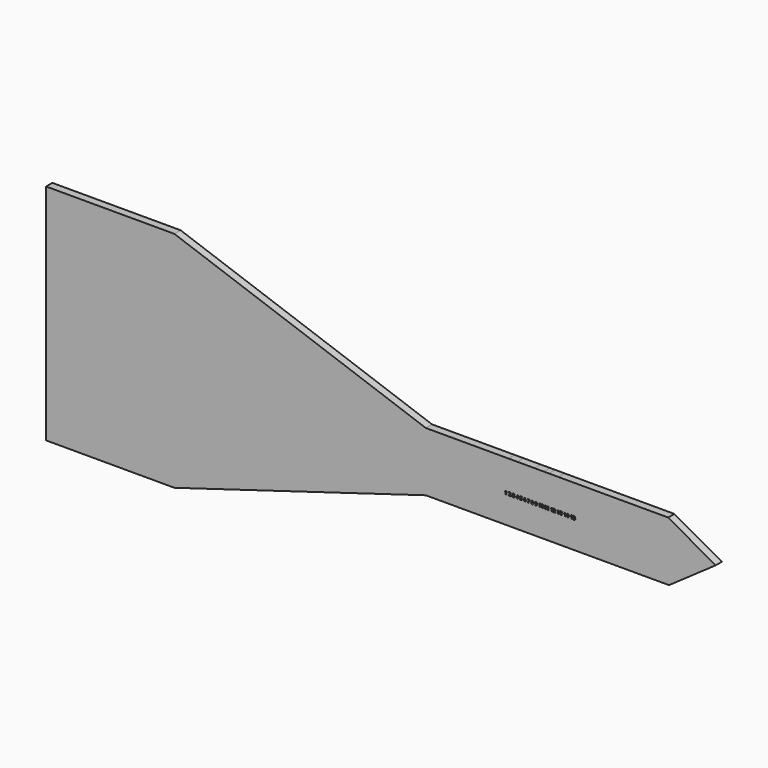
from build123d import *

# Parameters (mm, degrees)
F1_DEPTH = 1.42748
F7_DEPTH = 1.42748
F0_W     = 0.7037650794
F0_H     = 10.8203962445
F0_W_2   = 0.7917359471
F0_W_3   = 0.9236931801
F8_DEPTH = 1.42748


# Not quite as in the source:
# - the program builds the solid bodies; features that only make, move or delete a surface that nothing else refers to are left out


with BuildPart() as f1:
    # F0 (on Front) → F1 (new body)
    with BuildSketch(Plane.XZ):
        Polygon((0, 29.5358654112), (-45.9049940109, 45.8104424179), (-69.3307071924, 45.8104424179), (-69.3307071924, 4.9920389429), (-45.9049940109, 4.9920389429), (0, 18.7154691666), (14.3839064986, 18.7154691666), (14.3839064986, 29.5358654112), align=None)
    extrude(amount=F1_DEPTH)


with BuildPart() as f7:
    # F0 (on Front) → F7 (new body)
    with BuildSketch(Plane.XZ):
        Polygon((44.2517474294, 29.5358654112), (27.3507699184, 29.5358654112), (27.3507699184, 18.7154691666), (44.4178134203, 18.7154691666), (52.930470556, 24.6695391834), align=None)
    extrude(amount=F7_DEPTH)


with BuildPart() as f8:
    # F0 (on Front) → F8 (new body)
    with BuildSketch(Plane.XZ):
        Polygon((0, 29.5358654112), (-45.9049940109, 45.8104424179), (-69.3307071924, 45.8104424179), (-69.3307071924, 4.9920389429), (-45.9049940109, 4.9920389429), (0, 18.7154691666), (14.3839064986, 18.7154691666), (14.3839064986, 29.5358654112), align=None)
        with Locations((14.7357890382, 24.1256672889)):
            Rectangle(F0_W, F0_H)
        with BuildLine():
            Line((14.7264703071, 24.1856664079), (14.7264703071, 23.5936943802))
            Line((14.7264703071, 23.5936943802), (14.601312728, 23.5936943802))
            Line((14.601312728, 23.5936943802), (14.601312728, 23.9362581887))
            Line((14.601312728, 23.9362581887), (14.6026083551, 23.9924884054))
            Line((14.6026083551, 23.9924884054), (14.6045517958, 24.0540306932))
            add(Edge.make_bspline(
                [(14.6045517958, 24.0540306932), (14.5734567451, 24.0229356425), (14.5612778502, 24.0132184392)],
                knots=[0, 0, 0, 1, 1, 1], degree=2))
            Line((14.5612778502, 24.0132184392), (14.4932574268, 23.9585429751))
            Line((14.4932574268, 23.9585429751), (14.4328812034, 24.0338189103))
            Line((14.4328812034, 24.0338189103), (14.6235975144, 24.1856664079))
            Line((14.6235975144, 24.1856664079), (14.7264703071, 24.1856664079))
        make_face(mode=Mode.SUBTRACT)
        with BuildLine():
            Line((15.8354230225, 29.5358654112), (15.0876715779, 29.5358654112))
            Line((15.0876715779, 29.5358654112), (15.0876715779, 18.7154691666))
            Line((15.0876715779, 18.7154691666), (15.8354230225, 18.7154691666))
            Line((15.8354230225, 18.7154691666), (15.8354230225, 23.6024215287))
            add(Edge.make_bspline(
                [(15.8354230225, 23.6024215287), (15.8134077009, 23.6087806021), (15.793030546, 23.6175339191)],
                knots=[0.7264758514, 0.7264758514, 0.7264758514, 1, 1, 1], degree=2))
            Line((15.793030546, 23.6175339191), (15.793030546, 23.7240344677))
            add(Edge.make_bspline(
                [(15.793030546, 23.7240344677), (15.8130388008, 23.7139170861), (15.8354230225, 23.7059776741)],
                knots=[0, 0, 0, 0.5827513749, 0.5827513749, 0.5827513749], degree=2))
            Line((15.8354230225, 23.7059776741), (15.8354230225, 24.0738741563))
            Line((15.8354230225, 24.0738741563), (15.7938079223, 24.135784764))
            add(Edge.make_bspline(
                [(15.7938079223, 24.135784764), (15.8136756548, 24.1500895314), (15.8354230225, 24.1608846064)],
                knots=[0, 0, 0, 0.2453512407, 0.2453512407, 0.2453512407], degree=2))
            Line((15.8354230225, 24.1608846064), (15.8354230225, 29.5358654112))
        make_face()
        with BuildLine():
            Line((15.5196532253, 23.6990288644), (15.5196532253, 23.5936943802))
            Line((15.5196532253, 23.5936943802), (15.1058299256, 23.5936943802))
            Line((15.1058299256, 23.5936943802), (15.1058299256, 23.6807605222))
            Line((15.1058299256, 23.6807605222), (15.2544383554, 23.8309237045))
            add(Edge.make_bspline(
                [(15.2544383554, 23.8309237045), (15.3205153381, 23.8985554398), (15.3407271211, 23.9246623261)],
                knots=[0, 0, 0, 1, 1, 1], degree=2))
            add(Edge.make_bspline(
                [(15.3407271211, 23.9246623261), (15.360938904, 23.9507692124), (15.3698787311, 23.9730539987)],
                knots=[0, 0, 0, 1, 1, 1], degree=2))
            add(Edge.make_bspline(
                [(15.3698787311, 23.9730539987), (15.3788185582, 23.9953387851), (15.3788185582, 24.0191783239)],
                knots=[0, 0, 0, 1, 1, 1], degree=2))
            add(Edge.make_bspline(
                [(15.3788185582, 24.0191783239), (15.3788185582, 24.0548080695), (15.3591250261, 24.0722342542)],
                knots=[0, 0, 0, 1, 1, 1], degree=2))
            add(Edge.make_bspline(
                [(15.3591250261, 24.0722342542), (15.339431494, 24.0896604388), (15.306652128, 24.0896604388)],
                knots=[0, 0, 0, 1, 1, 1], degree=2))
            add(Edge.make_bspline(
                [(15.306652128, 24.0896604388), (15.2723180095, 24.0896604388), (15.2399273317, 24.0738537881)],
                knots=[0, 0, 0, 1, 1, 1], degree=2))
            add(Edge.make_bspline(
                [(15.2399273317, 24.0738537881), (15.2075366539, 24.0580471373), (15.1722955965, 24.0288955273)],
                knots=[0, 0, 0, 1, 1, 1], degree=2))
            Line((15.1722955965, 24.0288955273), (15.1042751731, 24.1094835337))
            add(Edge.make_bspline(
                [(15.1042751731, 24.1094835337), (15.1479378067, 24.1467975945), (15.1767007286, 24.1621507758)],
                knots=[0, 0, 0, 1, 1, 1], degree=2))
            add(Edge.make_bspline(
                [(15.1767007286, 24.1621507758), (15.2054636505, 24.1775039571), (15.2394738622, 24.1857959706)],
                knots=[0, 0, 0, 1, 1, 1], degree=2))
            add(Edge.make_bspline(
                [(15.2394738622, 24.1857959706), (15.2734840739, 24.1940879841), (15.3155919551, 24.1940879841)],
                knots=[0, 0, 0, 1, 1, 1], degree=2))
            add(Edge.make_bspline(
                [(15.3155919551, 24.1940879841), (15.3710447955, 24.1940879841), (15.4135413648, 24.1738762011)],
                knots=[0, 0, 0, 1, 1, 1], degree=2))
            add(Edge.make_bspline(
                [(15.4135413648, 24.1738762011), (15.4560379341, 24.1536644182), (15.4795535662, 24.117192515)],
                knots=[0, 0, 0, 1, 1, 1], degree=2))
            add(Edge.make_bspline(
                [(15.4795535662, 24.117192515), (15.5030691983, 24.0807206118), (15.5030691983, 24.0338189103)],
                knots=[0, 0, 0, 1, 1, 1], degree=2))
            add(Edge.make_bspline(
                [(15.5030691983, 24.0338189103), (15.5030691983, 23.9928770935), (15.4886877373, 23.9570530039)],
                knots=[0, 0, 0, 1, 1, 1], degree=2))
            add(Edge.make_bspline(
                [(15.4886877373, 23.9570530039), (15.4743062764, 23.9212289142), (15.4441181646, 23.8835909466)],
                knots=[0, 0, 0, 1, 1, 1], degree=2))
            add(Edge.make_bspline(
                [(15.4441181646, 23.8835909466), (15.4139300529, 23.845952979), (15.3378767414, 23.7762482403)],
                knots=[0, 0, 0, 1, 1, 1], degree=2))
            Line((15.3378767414, 23.7762482403), (15.2616938672, 23.704600061))
            Line((15.2616938672, 23.704600061), (15.2616938672, 23.6990288644))
            Line((15.2616938672, 23.6990288644), (15.5196532253, 23.6990288644))
        make_face(mode=Mode.SUBTRACT)
        with BuildLine():
            Line((16.7151298374, 29.5358654112), (15.8354230225, 29.5358654112))
            Line((15.8354230225, 29.5358654112), (15.8354230225, 24.1608846064))
            add(Edge.make_bspline(
                [(15.8354230225, 24.1608846064), (15.9023133469, 24.1940879841), (15.9869859248, 24.1940879841)],
                knots=[0.2453512407, 0.2453512407, 0.2453512407, 1, 1, 1], degree=2))
            add(Edge.make_bspline(
                [(15.9869859248, 24.1940879841), (16.078845887, 24.1940879841), (16.1320961613, 24.1568387046)],
                knots=[0, 0, 0, 1, 1, 1], degree=2))
            add(Edge.make_bspline(
                [(16.1320961613, 24.1568387046), (16.1853464357, 24.1195894251), (16.1853464357, 24.053253317)],
                knots=[0, 0, 0, 1, 1, 1], degree=2))
            add(Edge.make_bspline(
                [(16.1853464357, 24.053253317), (16.1853464357, 23.9978004766), (16.1517249121, 23.9589316632)],
                knots=[0, 0, 0, 1, 1, 1], degree=2))
            add(Edge.make_bspline(
                [(16.1517249121, 23.9589316632), (16.1181033885, 23.9200628498), (16.057338477, 23.9054222634)],
                knots=[0, 0, 0, 1, 1, 1], degree=2))
            Line((16.057338477, 23.9054222634), (16.057338477, 23.9030901346))
            add(Edge.make_bspline(
                [(16.057338477, 23.9030901346), (16.129116219, 23.8941503076), (16.165912029, 23.8594922823)],
                knots=[0, 0, 0, 1, 1, 1], degree=2))
            add(Edge.make_bspline(
                [(16.165912029, 23.8594922823), (16.202707839, 23.8248342571), (16.202707839, 23.7661423489)],
                knots=[0, 0, 0, 1, 1, 1], degree=2))
            add(Edge.make_bspline(
                [(16.202707839, 23.7661423489), (16.202707839, 23.6807605222), (16.140776863, 23.6331462258)],
                knots=[0, 0, 0, 1, 1, 1], degree=2))
            add(Edge.make_bspline(
                [(16.140776863, 23.6331462258), (16.078845887, 23.5855319294), (15.9639237622, 23.5855319294)],
                knots=[0, 0, 0, 1, 1, 1], degree=2))
            add(Edge.make_bspline(
                [(15.9639237622, 23.5855319294), (15.8938953715, 23.5855319294), (15.8354230225, 23.6024215287)],
                knots=[0, 0, 0, 0.7264758514, 0.7264758514, 0.7264758514], degree=2))
            Line((15.8354230225, 23.6024215287), (15.8354230225, 18.7154691666))
            Line((15.8354230225, 18.7154691666), (16.7151298374, 18.7154691666))
            Line((16.7151298374, 18.7154691666), (16.7151298374, 23.7163902677))
            Line((16.7151298374, 23.7163902677), (16.464294953, 23.7163902677))
            Line((16.464294953, 23.7163902677), (16.464294953, 23.8034564097))
            Line((16.464294953, 23.8034564097), (16.7151298374, 24.1726993783))
            Line((16.7151298374, 24.1726993783), (16.7151298374, 29.5358654112))
        make_face()
        with BuildLine():
            Line((17.3749104142, 29.5358654112), (16.7151298374, 29.5358654112))
            Line((16.7151298374, 29.5358654112), (16.7151298374, 24.1726993783))
            Line((16.7151298374, 24.1726993783), (16.7239386263, 24.1856664079))
            Line((16.7239386263, 24.1856664079), (16.8392494393, 24.1856664079))
            Line((16.8392494393, 24.1856664079), (16.8392494393, 23.8135623012))
            Line((16.8392494393, 23.8135623012), (16.9105089305, 23.8135623012))
            Line((16.9105089305, 23.8135623012), (16.9105089305, 23.7163902677))
            Line((16.9105089305, 23.7163902677), (16.8392494393, 23.7163902677))
            Line((16.8392494393, 23.7163902677), (16.8392494393, 23.5936943802))
            Line((16.8392494393, 23.5936943802), (16.7169422399, 23.5936943802))
            Line((16.7169422399, 23.5936943802), (16.7169422399, 23.7163902677))
            Line((16.7169422399, 23.7163902677), (16.7151298374, 23.7163902677))
            Line((16.7151298374, 23.7163902677), (16.7151298374, 18.7154691666))
            Line((16.7151298374, 18.7154691666), (17.3749104142, 18.7154691666))
            Line((17.3749104142, 18.7154691666), (17.3749104142, 23.5869744932))
            add(Edge.make_bspline(
                [(17.3749104142, 23.5869744932), (17.3576506722, 23.5855319294), (17.3389728166, 23.5855319294)],
                knots=[0.8358078197, 0.8358078197, 0.8358078197, 1, 1, 1], degree=2))
            add(Edge.make_bspline(
                [(17.3389728166, 23.5855319294), (17.2401164679, 23.5855319294), (17.179481119, 23.6175339191)],
                knots=[0, 0, 0, 1, 1, 1], degree=2))
            Line((17.179481119, 23.6175339191), (17.179481119, 23.725718783))
            add(Edge.make_bspline(
                [(17.179481119, 23.725718783), (17.211353546, 23.7087460678), (17.2539148966, 23.6979923627)],
                knots=[0, 0, 0, 1, 1, 1], degree=2))
            add(Edge.make_bspline(
                [(17.2539148966, 23.6979923627), (17.2964762473, 23.6872386577), (17.3344381217, 23.6872386577)],
                knots=[0, 0, 0, 1, 1, 1], degree=2))
            add(Edge.make_bspline(
                [(17.3344381217, 23.6872386577), (17.3568681065, 23.6872386577), (17.3749104142, 23.6908330825)],
                knots=[0, 0, 0, 0.1956165889, 0.1956165889, 0.1956165889], degree=2))
            Line((17.3749104142, 23.6908330825), (17.3749104142, 23.8667758689))
            add(Edge.make_bspline(
                [(17.3749104142, 23.8667758689), (17.3552666296, 23.8706994568), (17.3304216776, 23.8706994568)],
                knots=[0.7906549678, 0.7906549678, 0.7906549678, 1, 1, 1], degree=2))
            add(Edge.make_bspline(
                [(17.3304216776, 23.8706994568), (17.3090438303, 23.8706994568), (17.283131288, 23.8664238874)],
                knots=[0, 0, 0, 1, 1, 1], degree=2))
            add(Edge.make_bspline(
                [(17.283131288, 23.8664238874), (17.2572187458, 23.8621483179), (17.2410234069, 23.8572249349)],
                knots=[0, 0, 0, 1, 1, 1], degree=2))
            Line((17.2410234069, 23.8572249349), (17.191141763, 23.8840444161))
            Line((17.191141763, 23.8840444161), (17.2134265494, 24.1856664079))
            Line((17.2134265494, 24.1856664079), (17.3749104142, 24.1856664079))
            Line((17.3749104142, 24.1856664079), (17.3749104142, 29.5358654112))
        make_face()
        with BuildLine():
            Line((18.2546172291, 29.5358654112), (17.3749104142, 29.5358654112))
            Line((17.3749104142, 29.5358654112), (17.3749104142, 24.1856664079))
            Line((17.3749104142, 24.1856664079), (17.5344829478, 24.1856664079))
            Line((17.5344829478, 24.1856664079), (17.5344829478, 24.0795545474))
            Line((17.5344829478, 24.0795545474), (17.3749104142, 24.0795545474))
            Line((17.3749104142, 24.0795545474), (17.3749104142, 23.9717056243))
            add(Edge.make_bspline(
                [(17.3749104142, 23.9717056243), (17.3810481704, 23.9718879343), (17.3875588333, 23.9718879343)],
                knots=[0.8211706231, 0.8211706231, 0.8211706231, 1, 1, 1], degree=2))
            add(Edge.make_bspline(
                [(17.3875588333, 23.9718879343), (17.4733293481, 23.9718879343), (17.5241827123, 23.9236906057)],
                knots=[0, 0, 0, 1, 1, 1], degree=2))
            add(Edge.make_bspline(
                [(17.5241827123, 23.9236906057), (17.5750360765, 23.8754932772), (17.5750360765, 23.791666203)],
                knots=[0, 0, 0, 1, 1, 1], degree=2))
            add(Edge.make_bspline(
                [(17.5750360765, 23.791666203), (17.5750360765, 23.6925507289), (17.5138824768, 23.6390413291)],
                knots=[0, 0, 0, 1, 1, 1], degree=2))
            add(Edge.make_bspline(
                [(17.5138824768, 23.6390413291), (17.4627698199, 23.5943177544), (17.3749104142, 23.5869744932)],
                knots=[0, 0, 0, 0.8358078197, 0.8358078197, 0.8358078197], degree=2))
            Line((17.3749104142, 23.5869744932), (17.3749104142, 18.7154691666))
            Line((17.3749104142, 18.7154691666), (18.2546172291, 18.7154691666))
            Line((18.2546172291, 18.7154691666), (18.2546172291, 23.6896289949))
            add(Edge.make_bspline(
                [(18.2546172291, 23.6896289949), (18.2419338437, 23.66228672), (18.2212300988, 23.6408552071)],
                knots=[0.6126131022, 0.6126131022, 0.6126131022, 1, 1, 1], degree=2))
            add(Edge.make_bspline(
                [(18.2212300988, 23.6408552071), (18.1677854804, 23.5855319294), (18.0730751385, 23.5855319294)],
                knots=[0, 0, 0, 1, 1, 1], degree=2))
            add(Edge.make_bspline(
                [(18.0730751385, 23.5855319294), (18.0075164066, 23.5855319294), (17.9586712644, 23.6159143852)],
                knots=[0, 0, 0, 1, 1, 1], degree=2))
            add(Edge.make_bspline(
                [(17.9586712644, 23.6159143852), (17.9098261223, 23.646296841), (17.8833305479, 23.704600061)],
                knots=[0, 0, 0, 1, 1, 1], degree=2))
            add(Edge.make_bspline(
                [(17.8833305479, 23.704600061), (17.8568349734, 23.7629032811), (17.8568349734, 23.8451756027)],
                knots=[0, 0, 0, 1, 1, 1], degree=2))
            add(Edge.make_bspline(
                [(17.8568349734, 23.8451756027), (17.8568349734, 24.0208626392), (17.9311391883, 24.1066979354)],
                knots=[0, 0, 0, 1, 1, 1], degree=2))
            add(Edge.make_bspline(
                [(17.9311391883, 24.1066979354), (18.0054434032, 24.1925332316), (18.1536631449, 24.1925332316)],
                knots=[0, 0, 0, 1, 1, 1], degree=2))
            add(Edge.make_bspline(
                [(18.1536631449, 24.1925332316), (18.2041926023, 24.1925332316), (18.2329555241, 24.1864437841)],
                knots=[0, 0, 0, 1, 1, 1], degree=2))
            Line((18.2329555241, 24.1864437841), (18.2329555241, 24.0864213711))
            add(Edge.make_bspline(
                [(18.2329555241, 24.0864213711), (18.1969370904, 24.0945838219), (18.161696033, 24.0945838219)],
                knots=[0, 0, 0, 1, 1, 1], degree=2))
            add(Edge.make_bspline(
                [(18.161696033, 24.0945838219), (18.0973033655, 24.0945838219), (18.0566206741, 24.0751494152)],
                knots=[0, 0, 0, 1, 1, 1], degree=2))
            add(Edge.make_bspline(
                [(18.0566206741, 24.0751494152), (18.0159379828, 24.0557150085), (17.9957261999, 24.0176235714)],
                knots=[0, 0, 0, 1, 1, 1], degree=2))
            add(Edge.make_bspline(
                [(17.9957261999, 24.0176235714), (17.9755144169, 23.9795321343), (17.971886661, 23.9095682702)],
                knots=[0, 0, 0, 1, 1, 1], degree=2))
            Line((17.971886661, 23.9095682702), (17.9770691694, 23.9095682702))
            add(Edge.make_bspline(
                [(17.9770691694, 23.9095682702), (18.0172336099, 23.9783660699), (18.1054658163, 23.9783660699)],
                knots=[0, 0, 0, 1, 1, 1], degree=2))
            add(Edge.make_bspline(
                [(18.1054658163, 23.9783660699), (18.1847581956, 23.9783660699), (18.2297164564, 23.9285492074)],
                knots=[0, 0, 0, 1, 1, 1], degree=2))
            add(Edge.make_bspline(
                [(18.2297164564, 23.9285492074), (18.2446455683, 23.9120067188), (18.2546172291, 23.8912711122)],
                knots=[0, 0, 0, 0.3320660476, 0.3320660476, 0.3320660476], degree=2))
            Line((18.2546172291, 23.8912711122), (18.2546172291, 29.5358654112))
        make_face()
        with BuildLine():
            Line((19.0463531762, 29.5358654112), (18.2546172291, 29.5358654112))
            Line((18.2546172291, 29.5358654112), (18.2546172291, 23.8912711122))
            add(Edge.make_bspline(
                [(18.2546172291, 23.8912711122), (18.2746747172, 23.849562495), (18.2746747172, 23.7908888267)],
                knots=[0.3320660476, 0.3320660476, 0.3320660476, 1, 1, 1], degree=2))
            add(Edge.make_bspline(
                [(18.2746747172, 23.7908888267), (18.2746747172, 23.7328680303), (18.2546172291, 23.6896289949)],
                knots=[0, 0, 0, 0.6126131022, 0.6126131022, 0.6126131022], degree=2))
            Line((18.2546172291, 23.6896289949), (18.2546172291, 18.7154691666))
            Line((18.2546172291, 18.7154691666), (19.0463531762, 18.7154691666))
            Line((19.0463531762, 18.7154691666), (19.0463531762, 29.5358654112))
        make_face()
        Polygon((18.7395457251, 23.5936943802), (18.6082986986, 23.5936943802), (18.8306283111, 24.0795545474), (18.5387235227, 24.0795545474), (18.5387235227, 24.1848890316), (18.9634300901, 24.1848890316), (18.9634300901, 24.1062444659), align=None, mode=Mode.SUBTRACT)
        with Locations((19.4422211498, 24.1256672889)):
            Rectangle(F0_W_2, F0_H)
        with BuildLine():
            add(Edge.make_bspline(
                [(19.3052165224, 24.1540531063), (19.3578189832, 24.1933106078), (19.4424234336, 24.1933106078)],
                knots=[0, 0, 0, 1, 1, 1], degree=2))
            add(Edge.make_bspline(
                [(19.4424234336, 24.1933106078), (19.5275461349, 24.1933106078), (19.5795655634, 24.1546361385)],
                knots=[0, 0, 0, 1, 1, 1], degree=2))
            add(Edge.make_bspline(
                [(19.5795655634, 24.1546361385), (19.631584992, 24.1159616692), (19.631584992, 24.0504029373)],
                knots=[0, 0, 0, 1, 1, 1], degree=2))
            add(Edge.make_bspline(
                [(19.631584992, 24.0504029373), (19.631584992, 24.0050559884), (19.606449826, 23.9696205869)],
                knots=[0, 0, 0, 1, 1, 1], degree=2))
            add(Edge.make_bspline(
                [(19.606449826, 23.9696205869), (19.58131466, 23.9341851853), (19.5254731315, 23.9063292024)],
                knots=[0, 0, 0, 1, 1, 1], degree=2))
            add(Edge.make_bspline(
                [(19.5254731315, 23.9063292024), (19.5918092397, 23.8706994568), (19.6207665056, 23.8320249875)],
                knots=[0, 0, 0, 1, 1, 1], degree=2))
            add(Edge.make_bspline(
                [(19.6207665056, 23.8320249875), (19.6497237716, 23.7933505182), (19.6497237716, 23.7470966303)],
                knots=[0, 0, 0, 1, 1, 1], degree=2))
            add(Edge.make_bspline(
                [(19.6497237716, 23.7470966303), (19.6497237716, 23.6742823866), (19.5926513973, 23.629907158)],
                knots=[0, 0, 0, 1, 1, 1], degree=2))
            add(Edge.make_bspline(
                [(19.5926513973, 23.629907158), (19.535579023, 23.5855319294), (19.4424234336, 23.5855319294)],
                knots=[0, 0, 0, 1, 1, 1], degree=2))
            add(Edge.make_bspline(
                [(19.4424234336, 23.5855319294), (19.3452514002, 23.5855319294), (19.2897985598, 23.6268624343)],
                knots=[0, 0, 0, 1, 1, 1], degree=2))
            add(Edge.make_bspline(
                [(19.2897985598, 23.6268624343), (19.2343457193, 23.6681929392), (19.2343457193, 23.7438575625)],
                knots=[0, 0, 0, 1, 1, 1], degree=2))
            add(Edge.make_bspline(
                [(19.2343457193, 23.7438575625), (19.2343457193, 23.7945165826), (19.2612947633, 23.8337740841)],
                knots=[0, 0, 0, 1, 1, 1], degree=2))
            add(Edge.make_bspline(
                [(19.2612947633, 23.8337740841), (19.2882438072, 23.8730315856), (19.3477130917, 23.9030901346)],
                knots=[0, 0, 0, 1, 1, 1], degree=2))
            add(Edge.make_bspline(
                [(19.3477130917, 23.9030901346), (19.2970540716, 23.9349625616), (19.2748340666, 23.9714344648)],
                knots=[0, 0, 0, 1, 1, 1], degree=2))
            add(Edge.make_bspline(
                [(19.2748340666, 23.9714344648), (19.2526140616, 24.007906368), (19.2526140616, 24.0511803136)],
                knots=[0, 0, 0, 1, 1, 1], degree=2))
            add(Edge.make_bspline(
                [(19.2526140616, 24.0511803136), (19.2526140616, 24.1147956048), (19.3052165224, 24.1540531063)],
                knots=[0, 0, 0, 1, 1, 1], degree=2))
        make_face(mode=Mode.SUBTRACT)
        Polygon((20.6738114357, 29.5358654112), (19.8380891234, 29.5358654112), (19.8380891234, 18.7154691666), (20.6738114357, 18.7154691666), (20.6738114357, 23.9812896834), (20.6316795601, 24.0338189103), (20.6738114357, 24.0673641265), align=None)
        with BuildLine():
            add(Edge.make_bspline(
                [(20.3121779142, 24.0724933796), (20.3384791446, 24.0139958155), (20.3384791446, 23.9330191209)],
                knots=[0, 0, 0, 1, 1, 1], degree=2))
            add(Edge.make_bspline(
                [(20.3384791446, 23.9330191209), (20.3384791446, 23.7581094608), (20.2648227432, 23.6718206951)],
                knots=[0, 0, 0, 1, 1, 1], degree=2))
            add(Edge.make_bspline(
                [(20.2648227432, 23.6718206951), (20.1911663419, 23.5855319294), (20.0417805358, 23.5855319294)],
                knots=[0, 0, 0, 1, 1, 1], degree=2))
            add(Edge.make_bspline(
                [(20.0417805358, 23.5855319294), (19.9890485123, 23.5855319294), (19.9619699057, 23.5912326887)],
                knots=[0, 0, 0, 1, 1, 1], degree=2))
            Line((19.9619699057, 23.5912326887), (19.9619699057, 23.6916437899))
            add(Edge.make_bspline(
                [(19.9619699057, 23.6916437899), (19.9960448987, 23.6832222137), (20.0332293969, 23.6832222137)],
                knots=[0, 0, 0, 1, 1, 1], degree=2))
            add(Edge.make_bspline(
                [(20.0332293969, 23.6832222137), (20.0959377491, 23.6832222137), (20.1364260964, 23.7016201187)],
                knots=[0, 0, 0, 1, 1, 1], degree=2))
            add(Edge.make_bspline(
                [(20.1364260964, 23.7016201187), (20.1769144436, 23.7200180237), (20.1984218537, 23.7594698692)],
                knots=[0, 0, 0, 1, 1, 1], degree=2))
            add(Edge.make_bspline(
                [(20.1984218537, 23.7594698692), (20.2199292638, 23.7989217148), (20.2231683315, 23.8682377653)],
                knots=[0, 0, 0, 1, 1, 1], degree=2))
            Line((20.2231683315, 23.8682377653), (20.2182449485, 23.8682377653))
            add(Edge.make_bspline(
                [(20.2182449485, 23.8682377653), (20.1947940978, 23.8301463282), (20.1640229539, 23.8147931469)],
                knots=[0, 0, 0, 1, 1, 1], degree=2))
            add(Edge.make_bspline(
                [(20.1640229539, 23.8147931469), (20.1332518099, 23.7994399657), (20.0871274847, 23.7994399657)],
                knots=[0, 0, 0, 1, 1, 1], degree=2))
            add(Edge.make_bspline(
                [(20.0871274847, 23.7994399657), (20.0097785461, 23.7994399657), (19.9652089735, 23.8489977027)],
                knots=[0, 0, 0, 1, 1, 1], degree=2))
            add(Edge.make_bspline(
                [(19.9652089735, 23.8489977027), (19.9206394008, 23.8985554398), (19.9206394008, 23.9867876461)],
                knots=[0, 0, 0, 1, 1, 1], degree=2))
            add(Edge.make_bspline(
                [(19.9206394008, 23.9867876461), (19.9206394008, 24.0820162389), (19.9747318327, 24.1372747352)],
                knots=[0, 0, 0, 1, 1, 1], degree=2))
            add(Edge.make_bspline(
                [(19.9747318327, 24.1372747352), (20.0288242647, 24.1925332316), (20.1218502914, 24.1925332316)],
                knots=[0, 0, 0, 1, 1, 1], degree=2))
            add(Edge.make_bspline(
                [(20.1218502914, 24.1925332316), (20.187538586, 24.1925332316), (20.2367076349, 24.1617620876)],
                knots=[0, 0, 0, 1, 1, 1], degree=2))
            add(Edge.make_bspline(
                [(20.2367076349, 24.1617620876), (20.2858766838, 24.1309909437), (20.3121779142, 24.0724933796)],
                knots=[0, 0, 0, 1, 1, 1], degree=2))
        make_face(mode=Mode.SUBTRACT)
        with BuildLine():
            Line((21.5535182506, 29.5358654112), (20.6738114357, 29.5358654112))
            Line((20.6738114357, 29.5358654112), (20.6738114357, 24.0673641265))
            Line((20.6738114357, 24.0673641265), (20.822395871, 24.1856664079))
            Line((20.822395871, 24.1856664079), (20.9252686638, 24.1856664079))
            Line((20.9252686638, 24.1856664079), (20.9252686638, 23.5936943802))
            Line((20.9252686638, 23.5936943802), (20.8001110847, 23.5936943802))
            Line((20.8001110847, 23.5936943802), (20.8001110847, 23.9362581887))
            Line((20.8001110847, 23.9362581887), (20.8014067118, 23.9924884054))
            Line((20.8014067118, 23.9924884054), (20.8033501525, 24.0540306932))
            add(Edge.make_bspline(
                [(20.8033501525, 24.0540306932), (20.7722551018, 24.0229356425), (20.7600762069, 24.0132184392)],
                knots=[0, 0, 0, 1, 1, 1], degree=2))
            Line((20.7600762069, 24.0132184392), (20.6920557835, 23.9585429751))
            Line((20.6920557835, 23.9585429751), (20.6738114357, 23.9812896834))
            Line((20.6738114357, 23.9812896834), (20.6738114357, 18.7154691666))
            Line((20.6738114357, 18.7154691666), (21.5535182506, 18.7154691666))
            Line((21.5535182506, 18.7154691666), (21.5535182506, 29.5358654112))
        make_face()
        with BuildLine():
            add(Edge.make_bspline(
                [(21.4473416087, 24.1172572963), (21.4997497254, 24.0395196696), (21.4997497254, 23.8896156127)],
                knots=[0, 0, 0, 1, 1, 1], degree=2))
            add(Edge.make_bspline(
                [(21.4997497254, 23.8896156127), (21.4997497254, 23.73465861), (21.4489611426, 23.6600952697)],
                knots=[0, 0, 0, 1, 1, 1], degree=2))
            add(Edge.make_bspline(
                [(21.4489611426, 23.6600952697), (21.3981725598, 23.5855319294), (21.2924493874, 23.5855319294)],
                knots=[0, 0, 0, 1, 1, 1], degree=2))
            add(Edge.make_bspline(
                [(21.2924493874, 23.5855319294), (21.1899652828, 23.5855319294), (21.1379458543, 23.6624921799)],
                knots=[0, 0, 0, 1, 1, 1], degree=2))
            add(Edge.make_bspline(
                [(21.1379458543, 23.6624921799), (21.0859264257, 23.7394524303), (21.0859264257, 23.8896156127)],
                knots=[0, 0, 0, 1, 1, 1], degree=2))
            add(Edge.make_bspline(
                [(21.0859264257, 23.8896156127), (21.0859264257, 24.0463864933), (21.1365854458, 24.1206907082)],
                knots=[0, 0, 0, 1, 1, 1], degree=2))
            add(Edge.make_bspline(
                [(21.1365854458, 24.1206907082), (21.1872444659, 24.1949949231), (21.2924493874, 24.1949949231)],
                knots=[0, 0, 0, 1, 1, 1], degree=2))
            add(Edge.make_bspline(
                [(21.2924493874, 24.1949949231), (21.394933492, 24.1949949231), (21.4473416087, 24.1172572963)],
                knots=[0, 0, 0, 1, 1, 1], degree=2))
        make_face(mode=Mode.SUBTRACT)
        with Locations((22.0153648406, 24.1256672889)):
            Rectangle(F0_W_3, F0_H)
        with BuildLine():
            Line((21.9074303589, 24.1854990162), (21.9074303589, 23.5739164054))
            Line((21.9074303589, 23.5739164054), (21.7781266158, 23.5739164054))
            Line((21.7781266158, 23.5739164054), (21.7781266158, 23.9278285137))
            Line((21.7781266158, 23.9278285137), (21.7794651639, 23.9859214997))
            Line((21.7794651639, 23.9859214997), (21.781472986, 24.0495025328))
            add(Edge.make_bspline(
                [(21.781472986, 24.0495025328), (21.7493478324, 24.0173773792), (21.7367654806, 24.0073382688)],
                knots=[0, 0, 0, 1, 1, 1], degree=2))
            Line((21.7367654806, 24.0073382688), (21.6664917072, 23.9508515404))
            Line((21.6664917072, 23.9508515404), (21.6041153674, 24.028621183))
            Line((21.6041153674, 24.028621183), (21.8011496425, 24.1854990162))
            Line((21.8011496425, 24.1854990162), (21.9074303589, 24.1854990162))
        make_face(mode=Mode.SUBTRACT)
        with BuildLine():
            Line((22.3964019669, 24.1854990162), (22.3964019669, 23.5739164054))
            Line((22.3964019669, 23.5739164054), (22.2670982238, 23.5739164054))
            Line((22.2670982238, 23.5739164054), (22.2670982238, 23.9278285137))
            Line((22.2670982238, 23.9278285137), (22.2684367719, 23.9859214997))
            Line((22.2684367719, 23.9859214997), (22.270444594, 24.0495025328))
            add(Edge.make_bspline(
                [(22.270444594, 24.0495025328), (22.2383194404, 24.0173773792), (22.2257370886, 24.0073382688)],
                knots=[0, 0, 0, 1, 1, 1], degree=2))
            Line((22.2257370886, 24.0073382688), (22.1554633152, 23.9508515404))
            Line((22.1554633152, 23.9508515404), (22.0930869754, 24.028621183))
            Line((22.0930869754, 24.028621183), (22.2901212505, 24.1854990162))
            Line((22.2901212505, 24.1854990162), (22.3964019669, 24.1854990162))
        make_face(mode=Mode.SUBTRACT)
        with BuildLine():
            Line((23.3129318804, 29.5358654112), (22.4772114307, 29.5358654112))
            Line((22.4772114307, 29.5358654112), (22.4772114307, 18.7154691666))
            Line((22.4772114307, 18.7154691666), (23.3129318804, 18.7154691666))
            Line((23.3129318804, 18.7154691666), (23.3129318804, 23.5739164054))
            Line((23.3129318804, 23.5739164054), (23.2773004482, 23.5739164054))
            Line((23.2773004482, 23.5739164054), (23.2773004482, 23.6638668354))
            Line((23.2773004482, 23.6638668354), (23.3129318804, 23.6998710463))
            Line((23.3129318804, 23.6998710463), (23.3129318804, 24.0626745936))
            Line((23.3129318804, 24.0626745936), (23.2756941905, 24.10679239))
            add(Edge.make_bspline(
                [(23.2756941905, 24.10679239), (23.2958496272, 24.1240172142), (23.3129318804, 24.1367124332)],
                knots=[0, 0, 0, 0.4468156133, 0.4468156133, 0.4468156133], degree=2))
            Line((23.3129318804, 24.1367124332), (23.3129318804, 29.5358654112))
        make_face()
        with BuildLine():
            Line((23.107974118, 24.1854990162), (23.107974118, 23.5739164054))
            Line((23.107974118, 23.5739164054), (22.978670375, 23.5739164054))
            Line((22.978670375, 23.5739164054), (22.978670375, 23.9278285137))
            Line((22.978670375, 23.9278285137), (22.980008923, 23.9859214997))
            Line((22.980008923, 23.9859214997), (22.9820167451, 24.0495025328))
            add(Edge.make_bspline(
                [(22.9820167451, 24.0495025328), (22.9498915916, 24.0173773792), (22.9373092398, 24.0073382688)],
                knots=[0, 0, 0, 1, 1, 1], degree=2))
            Line((22.9373092398, 24.0073382688), (22.8670354664, 23.9508515404))
            Line((22.8670354664, 23.9508515404), (22.8046591266, 24.028621183))
            Line((22.8046591266, 24.028621183), (23.0016934017, 24.1854990162))
            Line((23.0016934017, 24.1854990162), (23.107974118, 24.1854990162))
        make_face(mode=Mode.SUBTRACT)
        with BuildLine():
            Line((24.1926386952, 29.5358654112), (23.3129318804, 29.5358654112))
            Line((23.3129318804, 29.5358654112), (23.3129318804, 24.1367124332))
            add(Edge.make_bspline(
                [(23.3129318804, 24.1367124332), (23.3340807289, 24.1524298717), (23.3505190273, 24.1612043688)],
                knots=[0.4468156133, 0.4468156133, 0.4468156133, 1, 1, 1], degree=2))
            add(Edge.make_bspline(
                [(23.3505190273, 24.1612043688), (23.3802347943, 24.1770661633), (23.415371681, 24.185632871)],
                knots=[0, 0, 0, 1, 1, 1], degree=2))
            add(Edge.make_bspline(
                [(23.415371681, 24.185632871), (23.4505085677, 24.1941995786), (23.4940113798, 24.1941995786)],
                knots=[0, 0, 0, 1, 1, 1], degree=2))
            add(Edge.make_bspline(
                [(23.4940113798, 24.1941995786), (23.551301237, 24.1941995786), (23.5952056135, 24.1733182288)],
                knots=[0, 0, 0, 1, 1, 1], degree=2))
            add(Edge.make_bspline(
                [(23.5952056135, 24.1733182288), (23.63910999, 24.152436879), (23.6634046374, 24.1147567509)],
                knots=[0, 0, 0, 1, 1, 1], degree=2))
            add(Edge.make_bspline(
                [(23.6634046374, 24.1147567509), (23.6876992848, 24.0770766229), (23.6876992848, 24.028621183)],
                knots=[0, 0, 0, 1, 1, 1], degree=2))
            add(Edge.make_bspline(
                [(23.6876992848, 24.028621183), (23.6876992848, 23.9863230641), (23.6728414013, 23.9493122102)],
                knots=[0, 0, 0, 1, 1, 1], degree=2))
            add(Edge.make_bspline(
                [(23.6728414013, 23.9493122102), (23.6579835177, 23.9123013562), (23.6267953478, 23.8734165349)],
                knots=[0, 0, 0, 1, 1, 1], degree=2))
            add(Edge.make_bspline(
                [(23.6267953478, 23.8734165349), (23.5956071779, 23.8345317136), (23.5170344065, 23.7625178277)],
                knots=[0, 0, 0, 1, 1, 1], degree=2))
            Line((23.5170344065, 23.7625178277), (23.4383277803, 23.6884961198))
            Line((23.4383277803, 23.6884961198), (23.4383277803, 23.6827403631))
            Line((23.4383277803, 23.6827403631), (23.7048327, 23.6827403631))
            Line((23.7048327, 23.6827403631), (23.7048327, 23.5739164054))
            Line((23.7048327, 23.5739164054), (23.3129318804, 23.5739164054))
            Line((23.3129318804, 23.5739164054), (23.3129318804, 18.7154691666))
            Line((23.3129318804, 18.7154691666), (24.1926386952, 18.7154691666))
            Line((24.1926386952, 18.7154691666), (24.1926386952, 23.5739164054))
            Line((24.1926386952, 23.5739164054), (24.1792141341, 23.5739164054))
            Line((24.1792141341, 23.5739164054), (24.1792141341, 23.9278285137))
            Line((24.1792141341, 23.9278285137), (24.1805526822, 23.9859214997))
            Line((24.1805526822, 23.9859214997), (24.1825605043, 24.0495025328))
            add(Edge.make_bspline(
                [(24.1825605043, 24.0495025328), (24.1504353507, 24.0173773792), (24.1378529989, 24.0073382688)],
                knots=[0, 0, 0, 1, 1, 1], degree=2))
            Line((24.1378529989, 24.0073382688), (24.0675792255, 23.9508515404))
            Line((24.0675792255, 23.9508515404), (24.0052028857, 24.028621183))
            Line((24.0052028857, 24.028621183), (24.1926386952, 24.1778567596))
            Line((24.1926386952, 24.1778567596), (24.1926386952, 29.5358654112))
        make_face()
        Polygon((25.2043027431, 29.5358654112), (24.1926386952, 29.5358654112), (24.1926386952, 24.1778567596), (24.2022371608, 24.1854990162), (24.3085178771, 24.1854990162), (24.3085178771, 23.5739164054), (24.1926386952, 23.5739164054), (24.1926386952, 18.7154691666), (25.2043027431, 18.7154691666), align=None)
        with BuildLine():
            add(Edge.make_bspline(
                [(24.8265359781, 24.1557163217), (24.8815503036, 24.1172330649), (24.8815503036, 24.048699404)],
                knots=[0, 0, 0, 1, 1, 1], degree=2))
            add(Edge.make_bspline(
                [(24.8815503036, 24.048699404), (24.8815503036, 23.9914095468), (24.8468149813, 23.9512531048)],
                knots=[0, 0, 0, 1, 1, 1], degree=2))
            add(Edge.make_bspline(
                [(24.8468149813, 23.9512531048), (24.812079659, 23.9110966629), (24.7493017548, 23.8959710698)],
                knots=[0, 0, 0, 1, 1, 1], degree=2))
            Line((24.7493017548, 23.8959710698), (24.7493017548, 23.8935616833))
            add(Edge.make_bspline(
                [(24.7493017548, 23.8935616833), (24.8234573176, 23.8843257016), (24.8614720826, 23.8485195409)],
                knots=[0, 0, 0, 1, 1, 1], degree=2))
            add(Edge.make_bspline(
                [(24.8614720826, 23.8485195409), (24.8994868477, 23.8127133802), (24.8994868477, 23.7520771528)],
                knots=[0, 0, 0, 1, 1, 1], degree=2))
            add(Edge.make_bspline(
                [(24.8994868477, 23.7520771528), (24.8994868477, 23.6638668354), (24.8355042502, 23.614675194)],
                knots=[0, 0, 0, 1, 1, 1], degree=2))
            add(Edge.make_bspline(
                [(24.8355042502, 23.614675194), (24.7715216527, 23.5654835526), (24.6527924394, 23.5654835526)],
                knots=[0, 0, 0, 1, 1, 1], degree=2))
            add(Edge.make_bspline(
                [(24.6527924394, 23.5654835526), (24.5532044633, 23.5654835526), (24.4762379496, 23.5985456898)],
                knots=[0, 0, 0, 1, 1, 1], degree=2))
            Line((24.4762379496, 23.5985456898), (24.4762379496, 23.7085743407))
            add(Edge.make_bspline(
                [(24.4762379496, 23.7085743407), (24.5117094733, 23.6906377967), (24.5544091566, 23.6793270655)],
                knots=[0, 0, 0, 1, 1, 1], degree=2))
            add(Edge.make_bspline(
                [(24.5544091566, 23.6793270655), (24.5971088399, 23.6680163344), (24.6388715395, 23.6680163344)],
                knots=[0, 0, 0, 1, 1, 1], degree=2))
            add(Edge.make_bspline(
                [(24.6388715395, 23.6680163344), (24.7029879918, 23.6680163344), (24.7335068876, 23.6897677404)],
                knots=[0, 0, 0, 1, 1, 1], degree=2))
            add(Edge.make_bspline(
                [(24.7335068876, 23.6897677404), (24.7640257835, 23.7115191465), (24.7640257835, 23.7597068768)],
                knots=[0, 0, 0, 1, 1, 1], degree=2))
            add(Edge.make_bspline(
                [(24.7640257835, 23.7597068768), (24.7640257835, 23.8026742697), (24.7288888968, 23.8206777411)],
                knots=[0, 0, 0, 1, 1, 1], degree=2))
            add(Edge.make_bspline(
                [(24.7288888968, 23.8206777411), (24.6937520101, 23.8386812126), (24.6167854964, 23.8386812126)],
                knots=[0, 0, 0, 1, 1, 1], degree=2))
            Line((24.6167854964, 23.8386812126), (24.5703378786, 23.8386812126))
            Line((24.5703378786, 23.8386812126), (24.5703378786, 23.9378676242))
            Line((24.5703378786, 23.9378676242), (24.6175886253, 23.9378676242))
            add(Edge.make_bspline(
                [(24.6175886253, 23.9378676242), (24.6886655275, 23.9378676242), (24.7215268825, 23.9564734423)],
                knots=[0, 0, 0, 1, 1, 1], degree=2))
            add(Edge.make_bspline(
                [(24.7215268825, 23.9564734423), (24.7543882375, 23.9750792604), (24.7543882375, 24.0201883302)],
                knots=[0, 0, 0, 1, 1, 1], degree=2))
            add(Edge.make_bspline(
                [(24.7543882375, 24.0201883302), (24.7543882375, 24.0896589747), (24.6673826133, 24.0896589747)],
                knots=[0, 0, 0, 1, 1, 1], degree=2))
            add(Edge.make_bspline(
                [(24.6673826133, 24.0896589747), (24.6372652818, 24.0896589747), (24.6060771119, 24.0796198642)],
                knots=[0, 0, 0, 1, 1, 1], degree=2))
            add(Edge.make_bspline(
                [(24.6060771119, 24.0796198642), (24.574888942, 24.0695807538), (24.536874177, 24.0449514694)],
                knots=[0, 0, 0, 1, 1, 1], degree=2))
            Line((24.536874177, 24.0449514694), (24.4770410785, 24.1339649157))
            add(Edge.make_bspline(
                [(24.4770410785, 24.1339649157), (24.5607003325, 24.1941995786), (24.6766185949, 24.1941995786)],
                knots=[0, 0, 0, 1, 1, 1], degree=2))
            add(Edge.make_bspline(
                [(24.6766185949, 24.1941995786), (24.7715216527, 24.1941995786), (24.8265359781, 24.1557163217)],
                knots=[0, 0, 0, 1, 1, 1], degree=2))
        make_face(mode=Mode.SUBTRACT)
        Polygon((26.084009558, 29.5358654112), (25.2043027431, 29.5358654112), (25.2043027431, 18.7154691666), (26.084009558, 18.7154691666), (26.084009558, 23.7006769072), (26.0460871198, 23.7006769072), (26.0460871198, 23.5739164054), (25.9197281825, 23.5739164054), (25.9197281825, 23.7006769072), (25.6587113099, 23.7006769072), (25.6587113099, 23.7906273371), (25.926956342, 24.1854990162), (26.0460871198, 24.1854990162), (26.0460871198, 23.801068012), (26.084009558, 23.801068012), align=None)
        with BuildLine():
            Line((25.5090616363, 24.1854990162), (25.5090616363, 23.5739164054))
            Line((25.5090616363, 23.5739164054), (25.3797578932, 23.5739164054))
            Line((25.3797578932, 23.5739164054), (25.3797578932, 23.9278285137))
            Line((25.3797578932, 23.9278285137), (25.3810964413, 23.9859214997))
            Line((25.3810964413, 23.9859214997), (25.3831042634, 24.0495025328))
            add(Edge.make_bspline(
                [(25.3831042634, 24.0495025328), (25.3509791098, 24.0173773792), (25.338396758, 24.0073382688)],
                knots=[0, 0, 0, 1, 1, 1], degree=2))
            Line((25.338396758, 24.0073382688), (25.2681229846, 23.9508515404))
            Line((25.2681229846, 23.9508515404), (25.2057466448, 24.028621183))
            Line((25.2057466448, 24.028621183), (25.4027809199, 24.1854990162))
            Line((25.4027809199, 24.1854990162), (25.5090616363, 24.1854990162))
        make_face(mode=Mode.SUBTRACT)
        with BuildLine():
            Line((27.2276289761, 29.5358654112), (26.084009558, 29.5358654112))
            Line((26.084009558, 29.5358654112), (26.084009558, 23.801068012))
            Line((26.084009558, 23.801068012), (26.1197072633, 23.801068012))
            Line((26.1197072633, 23.801068012), (26.1197072633, 23.7006769072))
            Line((26.1197072633, 23.7006769072), (26.084009558, 23.7006769072))
            Line((26.084009558, 23.7006769072), (26.084009558, 18.7154691666))
            Line((26.084009558, 18.7154691666), (27.2276289761, 18.7154691666))
            Line((27.2276289761, 18.7154691666), (27.2276289761, 23.617027051))
            add(Edge.make_bspline(
                [(27.2276289761, 23.617027051), (27.1648177861, 23.5654835526), (27.0513367163, 23.5654835526)],
                knots=[0.0344051631, 0.0344051631, 0.0344051631, 1, 1, 1], degree=2))
            add(Edge.make_bspline(
                [(27.0513367163, 23.5654835526), (26.949205499, 23.5654835526), (26.8865614495, 23.5985456898)],
                knots=[0, 0, 0, 1, 1, 1], degree=2))
            Line((26.8865614495, 23.5985456898), (26.8865614495, 23.7103144532))
            add(Edge.make_bspline(
                [(26.8865614495, 23.7103144532), (26.9194897319, 23.6927794736), (26.9634610359, 23.6816695246)],
                knots=[0, 0, 0, 1, 1, 1], degree=2))
            add(Edge.make_bspline(
                [(26.9634610359, 23.6816695246), (27.0074323398, 23.6705595757), (27.0466517981, 23.6705595757)],
                knots=[0, 0, 0, 1, 1, 1], degree=2))
            add(Edge.make_bspline(
                [(27.0466517981, 23.6705595757), (27.1651133018, 23.6705595757), (27.1651133018, 23.7676043104)],
                knots=[0, 0, 0, 1, 1, 1], degree=2))
            add(Edge.make_bspline(
                [(27.1651133018, 23.7676043104), (27.1651133018, 23.8600979817), (27.0425022991, 23.8600979817)],
                knots=[0, 0, 0, 1, 1, 1], degree=2))
            add(Edge.make_bspline(
                [(27.0425022991, 23.8600979817), (27.020416256, 23.8600979817), (26.9936452947, 23.855680773)],
                knots=[0, 0, 0, 1, 1, 1], degree=2))
            add(Edge.make_bspline(
                [(26.9936452947, 23.855680773), (26.9668743334, 23.8512635644), (26.9501424826, 23.8461770818)],
                knots=[0, 0, 0, 1, 1, 1], degree=2))
            Line((26.9501424826, 23.8461770818), (26.8986083821, 23.8738850267))
            Line((26.8986083821, 23.8738850267), (26.9216314088, 24.1854990162))
            Line((26.9216314088, 24.1854990162), (27.2276289761, 24.1854990162))
            Line((27.2276289761, 24.1854990162), (27.2276289761, 29.5358654112))
        make_face()
        with BuildLine():
            Line((26.7096053954, 24.1854990162), (26.7096053954, 23.5739164054))
            Line((26.7096053954, 23.5739164054), (26.5803016524, 23.5739164054))
            Line((26.5803016524, 23.5739164054), (26.5803016524, 23.9278285137))
            Line((26.5803016524, 23.9278285137), (26.5816402004, 23.9859214997))
            Line((26.5816402004, 23.9859214997), (26.5836480225, 24.0495025328))
            add(Edge.make_bspline(
                [(26.5836480225, 24.0495025328), (26.551522869, 24.0173773792), (26.5389405172, 24.0073382688)],
                knots=[0, 0, 0, 1, 1, 1], degree=2))
            Line((26.5389405172, 24.0073382688), (26.4686667438, 23.9508515404))
            Line((26.4686667438, 23.9508515404), (26.406290404, 24.028621183))
            Line((26.406290404, 24.028621183), (26.6033246791, 24.1854990162))
            Line((26.6033246791, 24.1854990162), (26.7096053954, 24.1854990162))
        make_face(mode=Mode.SUBTRACT)
        with BuildLine():
            Line((27.3507699184, 29.5358654112), (27.2276289761, 29.5358654112))
            Line((27.2276289761, 29.5358654112), (27.2276289761, 24.1854990162))
            Line((27.2276289761, 24.1854990162), (27.2533236192, 24.1854990162))
            Line((27.2533236192, 24.1854990162), (27.2533236192, 24.0758719297))
            Line((27.2533236192, 24.0758719297), (27.2276289761, 24.0758719297))
            Line((27.2276289761, 24.0758719297), (27.2276289761, 23.9275391363))
            add(Edge.make_bspline(
                [(27.2276289761, 23.9275391363), (27.2354932751, 23.921658014), (27.2426821621, 23.9148445975)],
                knots=[0.8631678895, 0.8631678895, 0.8631678895, 1, 1, 1], degree=2))
            add(Edge.make_bspline(
                [(27.2426821621, 23.9148445975), (27.2952201737, 23.8650506095), (27.2952201737, 23.7784465497)],
                knots=[0, 0, 0, 1, 1, 1], degree=2))
            add(Edge.make_bspline(
                [(27.2952201737, 23.7784465497), (27.2952201737, 23.6760476228), (27.232040705, 23.6207655877)],
                knots=[0, 0, 0, 1, 1, 1], degree=2))
            add(Edge.make_bspline(
                [(27.232040705, 23.6207655877), (27.2298670051, 23.6188636003), (27.2276289761, 23.617027051)],
                knots=[0, 0, 0, 0.0344051631, 0.0344051631, 0.0344051631], degree=2))
            Line((27.2276289761, 23.617027051), (27.2276289761, 18.7154691666))
            Line((27.2276289761, 18.7154691666), (27.3507699184, 18.7154691666))
            Line((27.3507699184, 18.7154691666), (27.3507699184, 29.5358654112))
        make_face()
        Polygon((44.2517474294, 29.5358654112), (27.3507699184, 29.5358654112), (27.3507699184, 18.7154691666), (44.4178134203, 18.7154691666), (52.930470556, 24.6695391834), align=None)
    extrude(amount=F8_DEPTH)


solid = Compound([f1.part, f7.part, f8.part])
